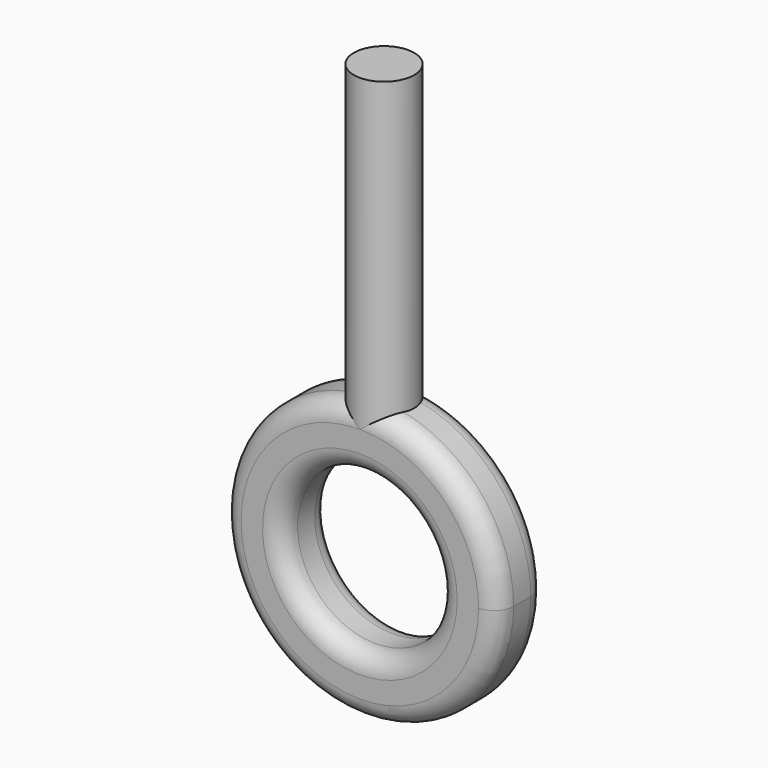
from build123d import *
from build123d import SkipClean  # not in build123d's __all__

# Parameters (mm, degrees)
F0_R          = 22.5425
F0_R_2        = 12.7
F1_DEPTH      = 9.8425
F2_R          = 3.175
F3_R          = 3.175
F5_R          = 4.92125
F6_DEPTH      = 50.8
F6_DEPTH_BACK = 3.175


with BuildPart() as f1:
    # F0 (on Front) → F1 (new body)
    with BuildSketch(Plane.XZ):
        Circle(F0_R)
        Circle(F0_R_2, mode=Mode.SUBTRACT)
    extrude(amount=F1_DEPTH)

    # F2
    f2_edges = [f1.edges().sort_by_distance(p)[0] for p in [
        (-22.5425, -9.8425, 0),
        (-22.5425, 0, 0),
    ]]
    fillet(f2_edges, radius=F2_R)

    # F3
    f3_edges = [f1.edges().sort_by_distance(p)[0] for p in [
        (-12.7, -9.8425, 0),
        (-12.7, 0, 0),
    ]]
    fillet(f3_edges, radius=F3_R)

    # F5 (on offset) → F6 (join, two sides)
    with BuildSketch(Plane.XY.offset(19.05)) as f6_sk:
        with Locations((0, -4.92125)):
            Circle(F5_R)
    with SkipClean():  # cleaning this boolean's faces spoils the solid; the shape is the same uncleaned
        extrude(amount=F6_DEPTH)
        extrude(f6_sk.sketch, amount=-F6_DEPTH_BACK)


solid = f1.part
